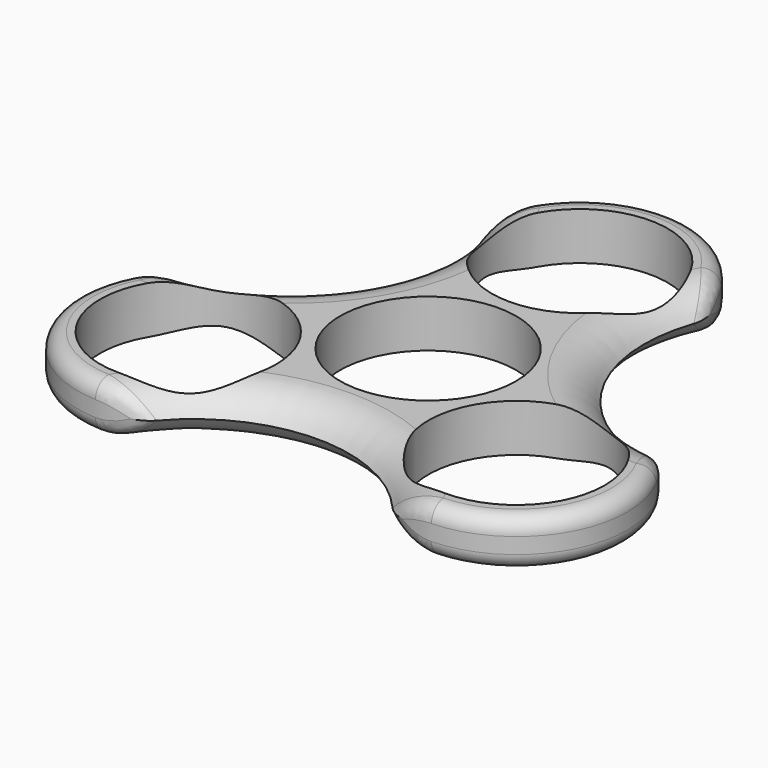
from build123d import *

# Parameters (mm, degrees)
F0_R         = 11.1
F1_DEPTH     = 6
F2_T2_ANGLE  = 184.5261330698
F2_T4_ANGLE  = 184.5261330698
F2_T6_ANGLE  = 184.5261330698
F2_T8_ANGLE  = 184.5261330698
F2_T10_ANGLE = 184.5261330698
F2_T12_ANGLE = 184.5261330698
F3_R         = 2


# Not quite as in the source:
# - a fillet or chamfer that OpenCascade refuses, or shapes differently, is made with other operations: its cross-section is extruded or revolved along the edge and cut away or added


with BuildPart() as f1:
    # F0 (on Top) → F1 (new body)
    with BuildSketch(Plane.XY):
        with BuildLine():
            ThreePointArc((27.6881337053, 0.1800560892), (15.7464316887, 9.0728231348), (13.9999690238, 23.8591486059))
            ThreePointArc((13.9999690238, 23.8591486059), (0.014725269, 37.8885913835), (-14, 23.8885991275))
            ThreePointArc((-14, 23.8885991275), (-15.7305111631, 9.100398294), (-27.6626133173, 0.1947545238))
            ThreePointArc((-27.6626133173, 0.1947545238), (-32.8198452862, -18.9315432347), (-13.6881337053, -24.0686552167))
            ThreePointArc((-13.6881337053, -24.0686552167), (-0.0159205256, -18.1732214287), (13.6626442935, -24.0539031297))
            ThreePointArc((13.6626442935, -24.0539031297), (32.8051200172, -18.9570481487), (27.6881337053, 0.1800560892))
        make_face()
        with Locations((-20.6881337053, -11.9442995638)):
            Circle(F0_R, mode=Mode.SUBTRACT)
        with Locations((20.6881337053, -11.9442995638)):
            Circle(F0_R, mode=Mode.SUBTRACT)
        Circle(F0_R, mode=Mode.SUBTRACT)
        with Locations((0, 23.8885991275)):
            Circle(F0_R, mode=Mode.SUBTRACT)
    extrude(amount=F1_DEPTH)

    # F2: fillet of radius 6 on 6 edges, made by hand

    # F2_s1 → F2_t2 (revolve, cut)
    with BuildSketch(Plane(origin=(31.2500144692, 19.7508361122, 0), x_dir=(0, 0, 1), z_dir=(0.8453180661, 0.5342633874, 0))):
        with BuildLine():
            ThreePointArc((0, 20.3116893746), (4.2426406871, 22.0690486875), (6, 26.3116893746))
            Line((6, 26.3116893746), (6, 20.3116893746))
            Line((6, 20.3116893746), (0, 20.3116893746))
        make_face()
    revolve(axis=Axis((32.0442915262, 18.4941212379, 6), (0, 0, -1)), revolution_arc=F2_T2_ANGLE, mode=Mode.SUBTRACT)

    # F2_s3 → F2_t4 (revolve, cut)
    with BuildSketch(Plane(origin=(31.2500144692, 19.7508361122, 0), x_dir=(0, 0, 1), z_dir=(0.8453180661, 0.5342633874, 0))):
        with BuildLine():
            ThreePointArc((6, 20.3116893746), (1.7573593129, 22.0690486875), (0, 26.3116893746))
            Line((0, 26.3116893746), (0, 20.3116893746))
            Line((0, 20.3116893746), (6, 20.3116893746))
        make_face()
    revolve(axis=Axis((32.0442915262, 18.4941212379, 0), (0, 0, -1)), revolution_arc=F2_T4_ANGLE, mode=Mode.SUBTRACT)

    # F2_s5 → F2_t6 (revolve, cut)
    with BuildSketch(Plane(origin=(1.4797185845, -36.9387244551, 0), x_dir=(0, 0, 1), z_dir=(0.0400266327, -0.9991986132, 0))):
        with BuildLine():
            ThreePointArc((0, 20.3116893746), (4.2426406871, 22.0690486875), (6, 26.3116893746))
            Line((6, 26.3116893746), (6, 20.3116893746))
            Line((6, 20.3116893746), (0, 20.3116893746))
        make_face()
    revolve(axis=Axis((-0.0057669504, -36.9982311269, 6), (0, 0, -1)), revolution_arc=F2_T6_ANGLE, mode=Mode.SUBTRACT)

    # F2_s7 → F2_t8 (revolve, cut)
    with BuildSketch(Plane(origin=(1.4797185845, -36.9387244551, 0), x_dir=(0, 0, 1), z_dir=(0.0400266327, -0.9991986132, 0))):
        with BuildLine():
            ThreePointArc((6, 20.3116893746), (1.7573593129, 22.0690486875), (0, 26.3116893746))
            Line((0, 26.3116893746), (0, 20.3116893746))
            Line((0, 20.3116893746), (6, 20.3116893746))
        make_face()
    revolve(axis=Axis((-0.0057669504, -36.9982311269, 0), (0, 0, -1)), revolution_arc=F2_T8_ANGLE, mode=Mode.SUBTRACT)

    # F2_s9 → F2_t10 (revolve, cut)
    with BuildSketch(Plane(origin=(-32.7297330538, 17.1878883429, 0), x_dir=(0, 0, 1), z_dir=(-0.8853446988, 0.4649352258, 0))):
        with BuildLine():
            ThreePointArc((0, 20.3116893746), (4.2426406871, 22.0690486875), (6, 26.3116893746))
            Line((6, 26.3116893746), (6, 20.3116893746))
            Line((6, 20.3116893746), (0, 20.3116893746))
        make_face()
    revolve(axis=Axis((-32.0385245758, 18.504109889, 6), (0, 0, -1)), revolution_arc=F2_T10_ANGLE, mode=Mode.SUBTRACT)

    # F2_s11 → F2_t12 (revolve, cut)
    with BuildSketch(Plane(origin=(-32.7297330538, 17.1878883429, 0), x_dir=(0, 0, 1), z_dir=(-0.8853446988, 0.4649352258, 0))):
        with BuildLine():
            ThreePointArc((6, 20.3116893746), (1.7573593129, 22.0690486875), (0, 26.3116893746))
            Line((0, 26.3116893746), (0, 20.3116893746))
            Line((0, 20.3116893746), (6, 20.3116893746))
        make_face()
    revolve(axis=Axis((-32.0385245758, 18.504109889, 0), (0, 0, -1)), revolution_arc=F2_T12_ANGLE, mode=Mode.SUBTRACT)

    # F3
    f3_edges = [f1.edges().sort_by_distance(p)[0] for p in [
        (0.005503, 37.888598, 0),
        (0.005503, 37.888598, 6),
        (32.809737, -18.949065, 0),
        (32.809737, -18.949065, 6),
        (-32.81524, -18.939533, 0),
        (-32.81524, -18.939533, 6),
    ]]
    fillet(f3_edges, radius=F3_R)


solid = f1.part
